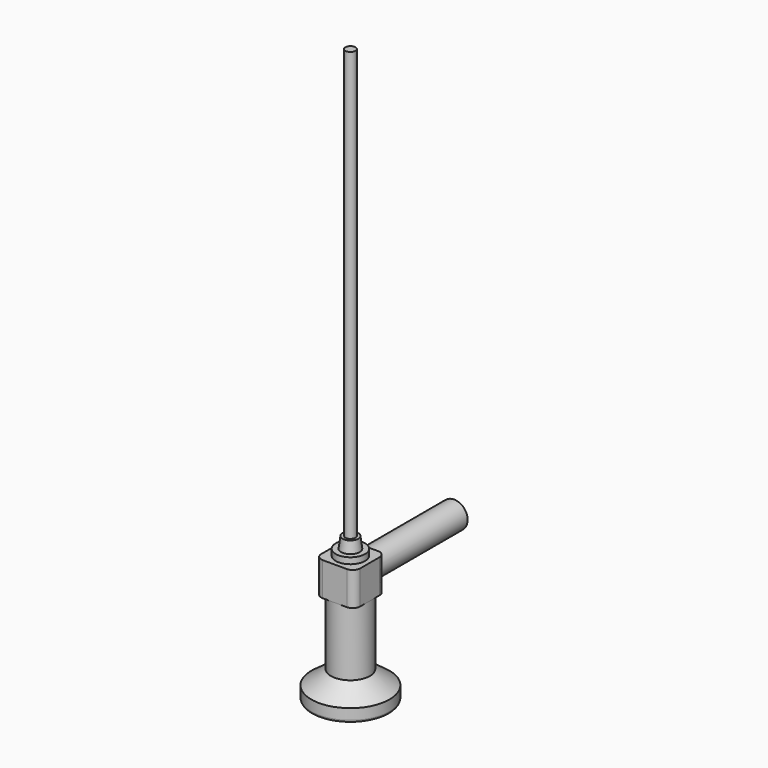
from build123d import *

# Parameters (mm, degrees)
F0_R      = 15.94
F1_DEPTH  = 5.34
F1_FACE_R = 15.94
F3_R      = 7.95
F5_DEPTH  = 27
F7_W      = 15.9
F7_H      = 15.9
F8_DEPTH  = 13.7
F10_R     = 5.5
F11_DEPTH = 45
F13_R     = 5.975
F14_DEPTH = 2.5
F16_R     = 3.8
F18_R     = 3.2
F21_R     = 2.05
F22_DEPTH = 175
F23_R     = 3
F24_R     = 1
F26_R     = 13
F27_DEPTH = 3
F28_R     = 2.99999


# Not quite as in the source:
# - a fillet or chamfer is up to 0.001 mm smaller than in the source, because OpenCascade refuses the exact size


with BuildPart() as f1:
    # F0 (on Top) → F1 (new body)
    with BuildSketch(Plane.XY):
        Circle(F0_R)
    extrude(amount=F1_DEPTH)

    # F1_face (on face) → F4 section 0
    with BuildSketch(Plane.XY.offset(5.34)):
        Circle(F1_FACE_R)
    # F3 (on offset) → F4 section 1
    with BuildSketch(Plane.XY.offset(11.18)):
        Circle(F3_R)
    loft()

    # F5 (add): a face of the model
    f5_faces = [f1.faces().sort_by_distance(p)[0] for p in [
        (0, 0, 11.18),
    ]]
    extrude(f5_faces, amount=F5_DEPTH)

    # F7 (on offset) → F8 (join)
    with BuildSketch(Plane.XY.offset(38.18)):
        Rectangle(F7_W, F7_H)
    extrude(amount=F8_DEPTH)

    # F10 (on offset) → F11 (join)
    with BuildSketch(Plane(origin=(0, 7.95, 0), x_dir=(-1, 0, 0), z_dir=(0, 1, 0))):
        with Locations((0, 45.03)):
            Circle(F10_R)
    extrude(amount=F11_DEPTH)

    # F13 (on offset) → F14 (join)
    with BuildSketch(Plane.XY.offset(51.88)):
        Circle(F13_R)
    extrude(amount=F14_DEPTH)

    # F16 (on offset) → F19 section 0
    with BuildSketch(Plane.XY.offset(54.38)):
        Circle(F16_R)
    # F18 (on offset) → F19 section 1
    with BuildSketch(Plane.XY.offset(58.97)):
        Circle(F18_R)
    loft()

    # F21 (on offset) → F22 (join)
    with BuildSketch(Plane.XY.offset(58.97)):
        Circle(F21_R)
    extrude(amount=F22_DEPTH)

    # F23
    f23_edges = [f1.edges().sort_by_distance(p)[0] for p in [
        (-7.95, -7.95, 45.03),
        (-7.95, 7.95, 45.03),
        (7.95, -7.95, 45.03),
        (7.95, 7.95, 45.03),
    ]]
    fillet(f23_edges, radius=F23_R)

    # F24
    f24_edges = [f1.edges().sort_by_distance(p)[0] for p in [
        (-15.94, 0, 0),
    ]]
    fillet(f24_edges, radius=F24_R)

    # F26 (on offset) → F27 (cut)
    with BuildSketch(Plane(origin=(0, 0, 0), x_dir=(1, 0, 0), z_dir=(0, 0, -1))):
        Circle(F26_R)
    extrude(amount=-F27_DEPTH, mode=Mode.SUBTRACT)

    # F28 (radius 3 in the source; OpenCascade refuses exactly that, so slightly less here)
    f28_edges = [f1.edges().sort_by_distance(p)[0] for p in [
        (-13, 0, 3),
    ]]
    fillet(f28_edges, radius=F28_R)


with BuildPart() as f29_1:
    # F29: copy of F1
    add(f1.part)


solid = f1.part
